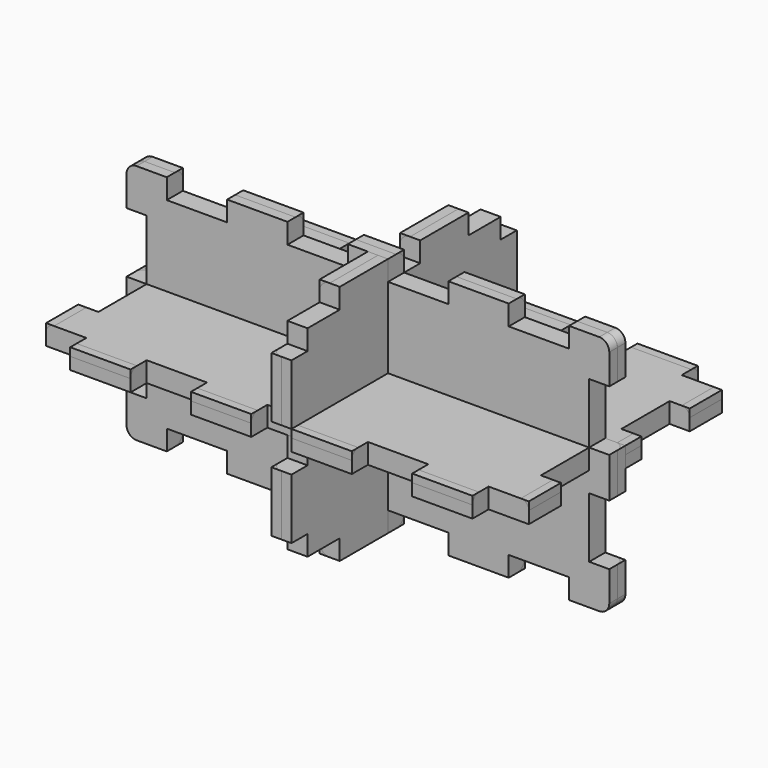
from build123d import *

# Parameters (mm, degrees)
F1_DEPTH      = 12.7
F4_DEPTH      = 12.7
F7_DEPTH      = 12.7
F9_R          = 6.35
F10_R         = 6.35
F11_R         = 6.35
F12_R         = 5.08
F13_R         = 6.35
F14_R         = 5.08
F15_T1_DEPTH  = 28.575
F15_T4_ANGLE  = 90
F15_T6_ANGLE  = 90
F15_T8_ANGLE  = 90
F15_T10_ANGLE = 90
F16_T1_DEPTH  = 22.225
F16_S5_W      = 6.35
F16_S5_H      = 6.35
F16_T6_DEPTH  = 6.35
F16_S11_W     = 6.35
F16_S11_H     = 6.35
F16_T12_DEPTH = 6.35
F16_S17_W     = 6.35
F16_S17_H     = 6.35
F16_T18_DEPTH = 6.35
F16_S23_W     = 6.35
F16_S23_H     = 6.35
F16_T24_DEPTH = 6.35


# Not quite as in the source:
# - a fillet or chamfer that OpenCascade refuses, or shapes differently, is made with other operations: its cross-section is extruded or revolved along the edge and cut away or added


with BuildPart() as f1:
    # F0 (on Top) → F1 (new body)
    with BuildSketch(Plane.XY):
        Polygon((88.9, -88.9), (127, -88.9), (127, -76.2), (152.4, -76.2), (152.4, -50.8), (139.7, -50.8), (139.7, -12.7), (152.4, -12.7), (152.4, 12.7), (139.7, 12.7), (139.7, 50.8), (152.4, 50.8), (152.4, 76.2), (127, 76.2), (127, 88.9), (88.9, 88.9), (88.9, 76.2), (50.8, 76.2), (50.8, 88.9), (12.7, 88.9), (12.7, 76.2), (-12.7, 76.2), (-12.7, 88.9), (-50.8, 88.9), (-50.8, 76.2), (-88.9, 76.2), (-88.9, 88.9), (-127, 88.9), (-127, 76.2), (-152.4, 76.2), (-152.4, 50.8), (-139.7, 50.8), (-139.7, 12.7), (-152.4, 12.7), (-152.4, -12.7), (-139.7, -12.7), (-139.7, -50.8), (-152.4, -50.8), (-152.4, -76.2), (-127, -76.2), (-127, -88.9), (-88.9, -88.9), (-88.9, -76.2), (-50.8, -76.2), (-50.8, -88.9), (-12.7, -88.9), (-12.7, -76.2), (12.7, -76.2), (12.7, -88.9), (50.8, -88.9), (50.8, -76.2), (88.9, -76.2), align=None)
    extrude(amount=F1_DEPTH)


with BuildPart() as f2_1:
    # F2: copy of F1
    add(f1.part)

    # F13
    f13_edges = [f2_1.edges().sort_by_distance(p)[0] for p in [
        (-152.4, 63.5, 0),
        (-107.95, 88.9, 0),
        (-31.75, 88.9, 0),
        (31.75, 88.9, 0),
        (31.75, -88.9, 0),
        (-31.75, -88.9, 0),
        (-107.95, -88.9, 0),
        (-152.4, -63.5, 0),
        (-152.4, 0, 0),
        (107.95, -88.9, 0),
        (152.4, -63.5, 0),
        (152.4, 0, 0),
        (152.4, 63.5, 0),
        (107.95, 88.9, 0),
    ]]
    fillet(f13_edges, radius=F13_R)


with BuildPart() as f4:
    # F3 (on Front) → F4 (new body)
    with BuildSketch(Plane.XZ):
        Polygon((152.4, 50.8), (152.4, 76.2), (127, 76.2), (127, 63.5), (88.9, 63.5), (88.9, 76.2), (50.8, 76.2), (50.8, 63.5), (12.7, 63.5), (12.7, 76.2), (-12.7, 76.2), (-12.7, 63.5), (-50.8, 63.5), (-50.8, 76.2), (-88.9, 76.2), (-88.9, 63.5), (-127, 63.5), (-127, 76.2), (-152.4, 76.2), (-152.4, 50.8), (-139.7, 50.8), (-139.7, 12.7), (-152.4, 12.7), (-152.4, -12.7), (-139.7, -12.7), (-139.7, -50.8), (-152.4, -50.8), (-152.4, -76.2), (-127, -76.2), (-127, -63.5), (-88.9, -63.5), (-88.9, -76.2), (-50.8, -76.2), (-50.8, -63.5), (-12.7, -63.5), (-12.7, -76.2), (12.7, -76.2), (12.7, -63.5), (50.8, -63.5), (50.8, -76.2), (88.9, -76.2), (88.9, -63.5), (127, -63.5), (127, -76.2), (152.4, -76.2), (152.4, -50.8), (139.7, -50.8), (139.7, -12.7), (152.4, -12.7), (152.4, 12.7), (139.7, 12.7), (139.7, 50.8), align=None)
    extrude(amount=F4_DEPTH)


with BuildPart() as f5_1:
    # F5: copy of F4
    add(f4.part)

    # F11
    f11_edges = [f5_1.edges().sort_by_distance(p)[0] for p in [
        (69.85, 0, 76.2),
        (0, 0, 76.2),
        (-69.85, 0, 76.2),
        (-139.7, 0, 76.2),
        (-152.4, 0, 63.5),
        (-152.4, 0, 0),
        (-139.7, 0, -76.2),
        (-152.4, 0, -63.5),
        (-69.85, 0, -76.2),
        (0, 0, -76.2),
        (69.85, 0, -76.2),
        (139.7, 0, -76.2),
        (152.4, 0, -63.5),
        (152.4, 0, 0),
        (152.4, 0, 63.5),
        (139.7, 0, 76.2),
    ]]
    fillet(f11_edges, radius=F11_R)

    # F16: fillet of radius 6.35 on 4 edges, made by hand

    # F16_s2 → F16_t1 (cut)
    with BuildSketch(Plane.XZ.offset(6.35)):
        with BuildLine():
            ThreePointArc((146.05, -76.2), (150.5401280605, -74.3401280605), (152.4, -69.85))
            Line((152.4, -69.85), (152.4, -76.2))
            Line((152.4, -76.2), (146.05, -76.2))
        make_face()
        with BuildLine():
            ThreePointArc((152.4, 69.85), (150.5401280605, 74.3401280605), (146.05, 76.2))
            Line((146.05, 76.2), (152.4, 76.2))
            Line((152.4, 76.2), (152.4, 69.85))
        make_face()
        with BuildLine():
            ThreePointArc((-146.05, 76.2), (-150.5401280605, 74.3401280605), (-152.4, 69.85))
            Line((-152.4, 69.85), (-152.4, 76.2))
            Line((-152.4, 76.2), (-146.05, 76.2))
        make_face()
        with BuildLine():
            ThreePointArc((-152.4, -69.85), (-150.5401280605, -74.3401280605), (-146.05, -76.2))
            Line((-146.05, -76.2), (-152.4, -76.2))
            Line((-152.4, -76.2), (-152.4, -69.85))
        make_face()
    extrude(amount=F16_T1_DEPTH, mode=Mode.SUBTRACT)


with BuildPart() as f7:
    # F6 (on Right) → F7 (new body)
    with BuildSketch(Plane.YZ):
        Polygon((50.8, 63.5), (50.8, 76.2), (12.7, 76.2), (12.7, 63.5), (-12.7, 63.5), (-12.7, 76.2), (-50.8, 76.2), (-50.8, 63.5), (-76.2, 63.5), (-76.2, 50.8), (-88.9, 50.8), (-88.9, 12.7), (-76.2, 12.7), (-76.2, -12.7), (-88.9, -12.7), (-88.9, -50.8), (-76.2, -50.8), (-76.2, -63.5), (-50.8, -63.5), (-50.8, -76.2), (-12.7, -76.2), (-12.7, -63.5), (12.7, -63.5), (12.7, -76.2), (50.8, -76.2), (50.8, -63.5), (76.2, -63.5), (76.2, -50.8), (88.9, -50.8), (88.9, -12.7), (76.2, -12.7), (76.2, 12.7), (88.9, 12.7), (88.9, 50.8), (76.2, 50.8), (76.2, 63.5), align=None)
    extrude(amount=F7_DEPTH)


with BuildPart() as f8_1:
    # F8: copy of F7
    add(f7.part)

    # F9
    f9_edges = [f8_1.edges().sort_by_distance(p)[0] for p in [
        (12.7, -31.75, 76.2),
        (12.7, 31.75, 76.2),
        (12.7, -88.9, 31.75),
        (12.7, -88.9, -31.75),
        (12.7, 88.9, 31.75),
        (12.7, 88.9, -31.75),
        (12.7, -31.75, -76.2),
        (12.7, 31.75, -76.2),
    ]]
    fillet(f9_edges, radius=F9_R)


with BuildPart() as f7_1:
    add(f7.part)

    # F10
    f10_edges = [f7_1.edges().sort_by_distance(p)[0] for p in [
        (0, 88.9, 31.75),
        (0, 88.9, -31.75),
        (0, 31.75, 76.2),
        (0, -31.75, 76.2),
        (0, -88.9, 31.75),
        (0, -88.9, -31.75),
        (0, 31.75, -76.2),
        (0, -31.75, -76.2),
    ]]
    fillet(f10_edges, radius=F10_R)


with BuildPart() as f1_1:
    add(f1.part)

    # F12
    f12_edges = [f1_1.edges().sort_by_distance(p)[0] for p in [
        (152.4, 63.5, 12.7),
        (152.4, 0, 12.7),
        (152.4, -63.5, 12.7),
        (107.95, 88.9, 12.7),
        (31.75, 88.9, 12.7),
        (-31.75, 88.9, 12.7),
        (107.95, -88.9, 12.7),
        (31.75, -88.9, 12.7),
        (-31.75, -88.9, 12.7),
        (-107.95, -88.9, 12.7),
        (-107.95, 88.9, 12.7),
        (-152.4, 63.5, 12.7),
        (-152.4, 0, 12.7),
        (-152.4, -63.5, 12.7),
    ]]
    fillet(f12_edges, radius=F12_R)


with BuildPart() as f4_1:
    add(f4.part)

    # F14
    f14_edges = [f4_1.edges().sort_by_distance(p)[0] for p in [
        (152.4, -12.7, 63.5),
        (139.7, -12.7, 76.2),
        (152.4, -12.7, 0),
        (152.4, -12.7, -63.5),
        (139.7, -12.7, -76.2),
        (69.85, -12.7, -76.2),
        (69.85, -12.7, 76.2),
        (0, -12.7, -76.2),
        (-69.85, -12.7, -76.2),
        (-139.7, -12.7, -76.2),
        (-152.4, -12.7, -63.5),
        (0, -12.7, 76.2),
        (-69.85, -12.7, 76.2),
        (-152.4, -12.7, 0),
        (-152.4, -12.7, 63.5),
        (-139.7, -12.7, 76.2),
    ]]
    fillet(f14_edges, radius=F14_R)

    # F15: fillet of radius 6.35 on 4 edges, made by hand

    # F15_s2 → F15_t1 (cut)
    with BuildSketch(Plane.XZ.offset(-15.875)):
        with BuildLine():
            ThreePointArc((-152.4, -69.85), (-150.5401280605, -74.3401280605), (-146.05, -76.2))
            Line((-146.05, -76.2), (-152.4, -76.2))
            Line((-152.4, -76.2), (-152.4, -69.85))
        make_face()
        with BuildLine():
            ThreePointArc((-146.05, 76.2), (-150.5401280605, 74.3401280605), (-152.4, 69.85))
            Line((-152.4, 69.85), (-152.4, 76.2))
            Line((-152.4, 76.2), (-146.05, 76.2))
        make_face()
        with BuildLine():
            ThreePointArc((152.4, 69.85), (150.5401280605, 74.3401280605), (146.05, 76.2))
            Line((146.05, 76.2), (152.4, 76.2))
            Line((152.4, 76.2), (152.4, 69.85))
        make_face()
        with BuildLine():
            ThreePointArc((146.05, -76.2), (150.5401280605, -74.3401280605), (152.4, -69.85))
            Line((152.4, -69.85), (152.4, -76.2))
            Line((152.4, -76.2), (146.05, -76.2))
        make_face()
    extrude(amount=F15_T1_DEPTH, mode=Mode.SUBTRACT)

    # F15_s3 → F15_t4 (revolve, cut)
    with BuildSketch(Plane.YZ.offset(146.05)):
        with BuildLine():
            ThreePointArc((-12.7, -71.12), (-11.2121024484, -74.7121024484), (-7.62, -76.2))
            Line((-7.62, -76.2), (-12.7, -76.2))
            Line((-12.7, -76.2), (-12.7, -71.12))
        make_face()
    revolve(axis=Axis((146.05, -12.7, -69.85), (0, -1, 0)), revolution_arc=F15_T4_ANGLE, mode=Mode.SUBTRACT)

    # F15_s5 → F15_t6 (revolve, cut)
    with BuildSketch(Plane.XY.offset(69.85)):
        with BuildLine():
            ThreePointArc((147.32, -12.7), (150.9121024484, -11.2121024484), (152.4, -7.62))
            Line((152.4, -7.62), (152.4, -12.7))
            Line((152.4, -12.7), (147.32, -12.7))
        make_face()
    revolve(axis=Axis((146.05, -12.7, 69.85), (0, -1, 0)), revolution_arc=F15_T6_ANGLE, mode=Mode.SUBTRACT)

    # F15_s7 → F15_t8 (revolve, cut)
    with BuildSketch(Plane.YZ.offset(-146.05)):
        with BuildLine():
            ThreePointArc((-12.7, 71.12), (-11.2121024484, 74.7121024484), (-7.62, 76.2))
            Line((-7.62, 76.2), (-12.7, 76.2))
            Line((-12.7, 76.2), (-12.7, 71.12))
        make_face()
    revolve(axis=Axis((-146.05, -12.7, 69.85), (0, -1, 0)), revolution_arc=F15_T8_ANGLE, mode=Mode.SUBTRACT)

    # F15_s9 → F15_t10 (revolve, cut)
    with BuildSketch(Plane.XY.offset(-69.85)):
        with BuildLine():
            ThreePointArc((-147.32, -12.7), (-150.9121024484, -11.2121024484), (-152.4, -7.62))
            Line((-152.4, -7.62), (-152.4, -12.7))
            Line((-152.4, -12.7), (-147.32, -12.7))
        make_face()
    revolve(axis=Axis((-146.05, -12.7, -69.85), (0, -1, 0)), revolution_arc=F15_T10_ANGLE, mode=Mode.SUBTRACT)


with BuildPart() as f16_tool4:
    # F16_s5 → F16_t6 (new body)
    with BuildSketch(Plane.YZ.offset(-146.05)):
        with Locations((-3.175, -73.025)):
            Rectangle(F16_S5_W, F16_S5_H)
    extrude(amount=-F16_T6_DEPTH)

    # F16_s7 → F16_t8 (revolve, cut)
    with BuildSketch(Plane(origin=(-146.05, -6.35, -69.85), x_dir=(0, -0.7071067812, 0.7071067812), z_dir=(0, -0.7071067812, -0.7071067812))):
        with BuildLine():
            ThreePointArc((0, -6.35), (6.35, 0), (0, 6.35))
            Line((0, 6.35), (0, -6.35))
        make_face()
    revolve(axis=Axis((-146.05, -6.35, -69.85), (-1, 0, 0)), mode=Mode.SUBTRACT)


with BuildPart() as f5_1_1:
    add(f5_1.part)

    # F16_t3: cut F16_tool4
    add(f16_tool4.part, mode=Mode.SUBTRACT)


with BuildPart() as f16_tool10:
    # F16_s11 → F16_t12 (new body)
    with BuildSketch(Plane.XY.offset(69.85)):
        with Locations((-149.225, -3.175)):
            Rectangle(F16_S11_W, F16_S11_H)
    extrude(amount=F16_T12_DEPTH)

    # F16_s13 → F16_t14 (revolve, cut)
    with BuildSketch(Plane(origin=(-146.05, -6.35, 69.85), x_dir=(0.7071067812, -0.7071067812, 0), z_dir=(-0.7071067812, -0.7071067812, 0))):
        with BuildLine():
            ThreePointArc((0, -6.35), (6.35, 0), (0, 6.35))
            Line((0, 6.35), (0, -6.35))
        make_face()
    revolve(axis=Axis((-146.05, -6.35, 69.85), (0, 0, 1)), mode=Mode.SUBTRACT)


with BuildPart() as f5_1_2:
    add(f5_1_1.part)

    # F16_t9: cut F16_tool10
    add(f16_tool10.part, mode=Mode.SUBTRACT)


with BuildPart() as f16_tool16:
    # F16_s17 → F16_t18 (new body)
    with BuildSketch(Plane.YZ.offset(146.05)):
        with Locations((-3.175, 73.025)):
            Rectangle(F16_S17_W, F16_S17_H)
    extrude(amount=F16_T18_DEPTH)

    # F16_s19 → F16_t20 (revolve, cut)
    with BuildSketch(Plane(origin=(146.05, -6.35, 69.85), x_dir=(0, -0.7071067812, -0.7071067812), z_dir=(0, -0.7071067812, 0.7071067812))):
        with BuildLine():
            ThreePointArc((0, -6.35), (6.35, 0), (0, 6.35))
            Line((0, 6.35), (0, -6.35))
        make_face()
    revolve(axis=Axis((146.05, -6.35, 69.85), (1, 0, 0)), mode=Mode.SUBTRACT)


with BuildPart() as f5_1_3:
    add(f5_1_2.part)

    # F16_t15: cut F16_tool16
    add(f16_tool16.part, mode=Mode.SUBTRACT)


with BuildPart() as f16_tool22:
    # F16_s23 → F16_t24 (new body)
    with BuildSketch(Plane.XY.offset(-69.85)):
        with Locations((149.225, -3.175)):
            Rectangle(F16_S23_W, F16_S23_H)
    extrude(amount=-F16_T24_DEPTH)

    # F16_s25 → F16_t26 (revolve, cut)
    with BuildSketch(Plane(origin=(146.05, -6.35, -69.85), x_dir=(-0.7071067812, -0.7071067812, 0), z_dir=(0.7071067812, -0.7071067812, 0))):
        with BuildLine():
            ThreePointArc((0, -6.35), (6.35, 0), (0, 6.35))
            Line((0, 6.35), (0, -6.35))
        make_face()
    revolve(axis=Axis((146.05, -6.35, -69.85), (0, 0, -1)), mode=Mode.SUBTRACT)


with BuildPart() as f5_1_4:
    add(f5_1_3.part)

    # F16_t21: cut F16_tool22
    add(f16_tool22.part, mode=Mode.SUBTRACT)


solid = Compound([f2_1.part, f8_1.part, f7_1.part, f1_1.part, f4_1.part, f5_1_4.part])
